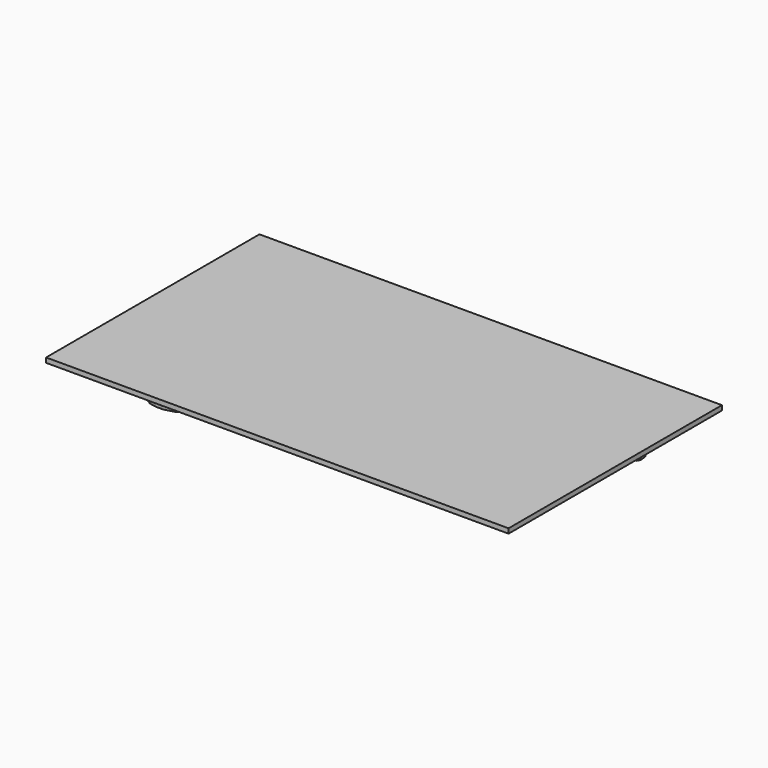
from build123d import *

# Parameters (mm, degrees)
F1_DEPTH = 2
F3_W     = 97.3806902766
F3_H     = 56.1529509723
F4_DEPTH = 1


with BuildPart() as f1:
    # F0 (on Top) → F1 (new body)
    with BuildSketch(Plane.XY):
        Polygon((23.6468666, -2.9716222), (23.3256315665, -2.7068344444), (23.2722166, -2.7745182), (23.0324406, -2.9523436), (22.6933506, -3.1164276), (22.3049846, -3.1880556), (22.1726506, -3.1880556), (21.7385646, -3.0351476), (21.4050626, -2.7651456), (21.2343746, -2.6602436), (20.8787746, -2.4037036), (20.5562335082, -2.1246834637), (20.5313026, -2.3142956), (20.5051406, -2.4204676), (20.2666346, -2.6328116), (20.1343006, -2.8172156), (19.8698866, -3.0818582), (18.9603126, -3.8385242), (17.8333146, -4.1403016), (17.7629566, -3.8880796), (17.8333146, -3.4788856), (18.0715666, -2.9233622), (18.4144666, -2.5787096), (19.4756786, -2.3211536), (20.5370916003, -2.1081244023), (20.5079346, -2.0829016), (20.2945746, -1.7849596), (20.2046131837, -1.7139919569), (19.3946526, -1.8390616), (18.9438026, -1.9973036), (18.4144666, -2.0496022), (17.9214526, -2.3005796), (17.5686466, -2.7110436), (17.2519086, -3.4527236), (17.1716446, -3.7432996), (17.2778166, -4.2464736), (17.5948086, -4.4585636), (18.0441346, -4.4806616), (18.4947306, -4.4049442), (18.5468006, -4.3785536), (19.2361566, -4.1403016), (19.6590666, -3.7694616), (19.3405506, -4.3262296), (19.0499746, -4.9078642), (18.6270646, -5.8862976), (18.5747406, -6.0983622), (18.7027566, -6.5380616), (19.0499746, -6.7598036), (19.5351146, -6.7791076), (20.0019666, -6.6015616), (20.5368906, -6.0846462), (21.1144866, -5.6493156), (21.3250526, -6.0722256), (21.4312246, -6.5477136), (21.6161366, -6.8080636), (21.8820746, -7.0506082), (22.0926406, -7.1044816), (22.7375466, -7.1623936), (23.2049066, -6.9444616), (23.3634026, -6.7074796), (23.3923586, -6.0681616), (23.3634026, -5.4892956), (23.3235246, -4.9739296), (23.2049066, -4.4585636), (23.3093006, -4.4585636), (23.8663226, -5.0925476), (23.9986566, -5.3846222), (24.8447306, -5.8862976), (25.3738126, -6.1245496), (25.5061466, -6.1783722), (25.9318506, -6.0750196), (26.2198866, -5.7539636), (26.2475726, -5.6754776), (26.1937246, -5.0262536), (25.9831586, -4.4585636), (25.6905506, -4.0313102), (25.3999746, -3.6648136), (25.1642626, -3.4816796), (25.1049691663, -3.4368495289), (24.4477286, -3.3727136), (24.3677186, -3.4527236), (24.2656106, -3.3823402), (23.9958626, -3.2129476), align=None)
        Polygon((20.4528166, -5.4892956), (20.2404726, -5.6754776), (19.9953626, -6.0282836), (19.7113906, -6.2830456), (19.1823086, -6.3368682), (19.2361566, -6.0186316), (19.8437246, -4.6955456), (20.7698086, -3.4003742), (20.9018886, -3.2045656), (21.1144866, -3.1080456), (21.0342226, -3.6373816), (20.9018886, -4.2203116), (20.7436466, -4.6432216), (20.6113126, -5.0925476), align=None, mode=Mode.SUBTRACT)
        Polygon((21.9603066, -4.4585636), (22.1726506, -3.8756082), (22.2249746, -3.5586416), (22.3832166, -3.3465516), (22.5155506, -3.4885376), (22.6478846, -3.6909756), (22.6631246, -4.1169336), (22.7497386, -4.7217076), (22.8521006, -5.3267356), (22.9125526, -5.7539636), (22.9554786, -6.0709302), (22.9402386, -6.3892176), (22.8602286, -6.5477136), (22.6577906, -6.7364102), (22.3573086, -6.7861942), (22.3311466, -6.7861942), (22.1878906, -6.5050416), (22.0664786, -6.2045596), (21.9864686, -5.4892956), (21.9082366, -4.8017176), align=None, mode=Mode.SUBTRACT)
        Polygon((24.6488966, -5.1613816), (24.1833146, -4.4585636), (24.0372646, -4.1306496), (23.8924846, -3.7432996), (23.8081566, -3.4842196), (23.7863126, -3.3465516), (23.9707166, -3.3727136), (24.1571526, -3.4003742), (24.6227346, -3.5642296), (24.9509026, -3.8494716), (25.2305566, -4.0864282), (25.4538226, -4.4049442), (25.7474466, -4.9271936), (25.7446526, -5.6493156), (25.6905506, -5.7016142), (25.2938026, -5.6493156), align=None, mode=Mode.SUBTRACT)
        Polygon((23.8233966, -2.3833836), (23.6172765796, -2.0582420765), (23.3634026, -2.6589736), (23.3256315665, -2.7068344444), (23.6468666, -2.9716222), (23.9958626, -3.2129476), (24.2656106, -3.3823402), (24.3677186, -3.4527236), (24.4477286, -3.3727136), (25.1049691663, -3.4368495289), (24.9509026, -3.3203642), (24.5800626, -3.0874716), (24.1309906, -2.8972256), (24.0509806, -2.8710636), (23.9448086, -2.7389836), align=None)
        Polygon((24.8185686, -1.4161516), (24.8035180213, -1.4201773166), (23.6539786, -1.9713956), (23.6172765796, -2.0582420765), (23.8233966, -2.3833836), (23.9448086, -2.7389836), (24.0509806, -2.8710636), (24.1309906, -2.8972256), (24.5800626, -3.0874716), (24.9509026, -3.3203642), (25.1049691663, -3.4368495289), (25.2676406, -3.4527236), (25.5582166, -3.5586416), (26.5122406, -3.3203642), (27.0413226, -3.1080456), (27.1736566, -3.0295596), (27.4065746, -2.6617422), (27.3842226, -2.2358096), (27.3583146, -2.1819616), (26.8813026, -1.7811496), (26.3260586, -1.5205456), (25.8393946, -1.4118336), (25.3738126, -1.3620496), (25.0746006, -1.3785596), align=None)
        Polygon((25.8863846, -2.9592016), (25.0570746, -2.7910536), (24.7344946, -2.6645616), (24.3956586, -2.5004776), (24.1528346, -2.3734776), (24.0509806, -2.2881082), (24.1833146, -2.1819616), (24.3153946, -2.0775676), (24.7507506, -1.8679922), (25.1894086, -1.8390616), (25.5488186, -1.8016982), (25.9290566, -1.8652236), (26.5107166, -2.0402042), (27.0136366, -2.5528016), (27.0136366, -2.6328116), (26.6966446, -2.8710636), align=None, mode=Mode.SUBTRACT)
        Polygon((25.1091446, 1.3359384), (24.5000526, 0.9130284), (24.2714526, 0.6592824), (24.0248186, 0.4639564), (24.1007646, 0.7517638), (24.1571526, 1.0974324), (24.2633246, 1.7329404), (24.3956586, 2.7911044), (24.3956586, 3.0034484), (24.1556286, 3.3948624), (23.7601506, 3.5066478), (23.2831386, 3.3839404), (22.8863906, 3.0819344), (22.5282506, 2.4550624), (22.0926406, 1.8650204), (21.7759026, 2.2096984), (21.5373966, 2.6328878), (21.2988906, 2.8353004), (20.9821526, 2.9775404), (20.7698086, 2.9775404), (20.1579226, 2.8726384), (19.7652386, 2.5266904), (19.6852286, 2.2358858), (19.8465186, 1.6255238), (20.0299066, 1.0712704), (20.2239626, 0.5864098), (20.4789786, 0.1192784), (20.3728066, 0.0931418), (19.6852286, 0.5421884), (19.4728846, 0.7806944), (18.5206386, 1.0192004), (17.9653946, 1.0974324), (17.8333146, 1.0974324), (17.4652686, 0.8840724), (17.2778166, 0.4901438), (17.2778166, 0.4098544), (17.5216566, -0.1812036), (17.8853846, -0.6744716), (18.2684166, -1.0079482), (18.6529726, -1.2838176), (18.9275466, -1.3981176), (19.1823086, -1.4943582), (19.6014086, -1.6170656), (20.0822306, -1.6805656), (20.1622406, -1.6805656), (20.2046131837, -1.7139919569), (20.7698086, -1.6267176), (21.2465666, -1.0453116), (21.3679786, -0.9584436), (21.6489026, -0.8591296), (22.0194886, -0.7986522), (22.4111566, -0.8329676), (22.5434906, -0.8591296), (22.9153466, -1.1334496), (23.0297911258, -1.2959904244), (23.2435146, -1.3691616), (23.4154726, -1.6805656), (23.4154726, -1.7328642), (23.4089527537, -1.7725239478), (23.4243429347, -1.7923627405), (23.7063026, -1.7067276), (23.8924846, -1.7328642), (23.9448086, -1.7067276), (24.3913406, -1.5304262), (24.8035180213, -1.4201773166), (24.9247406, -1.3620496), (25.3214886, -1.0714736), (25.8228846, -0.8591296), (26.2391906, -0.4814316), (26.4581386, 0.0131318), (26.5645646, 0.8068818), (26.5645646, 1.1253978), (26.3260586, 1.5744444), (25.9831586, 1.6806418), (25.5378966, 1.5716504), (25.1353066, 1.3621258), align=None)
        Polygon((19.0073026, 0.3715004), (19.6590666, -0.1715516), (19.8863966, -0.4483862), (20.1343006, -0.8068056), (20.2902566, -1.0288016), (20.3466446, -1.1514836), (20.1622406, -1.1776456), (19.9760586, -1.2035536), (19.4993006, -1.1761216), (19.1038226, -0.9912096), (18.7649866, -0.8428736), (18.4685686, -0.5944616), (18.0304186, -0.1784096), (17.8333146, 0.5160264), (17.8592226, 0.5962904), (18.2562246, 0.6745224), align=None, mode=Mode.SUBTRACT)
        Polygon((23.9186466, -0.8068056), (23.9986566, -0.5944616), (24.1833146, -0.2777236), (24.4766846, 0.2348484), (24.8239026, 0.7047484), (25.2610366, 1.0811764), (25.8228846, 1.3097764), (25.9552186, 1.1017504), (26.0090666, 0.6745224), (25.9290566, 0.0669544), (25.8091686, -0.1646936), (25.6905506, -0.3577336), (24.7355106, -0.9058656), (23.7601506, -1.4161516), (23.7339886, -1.2035536), (23.7339886, -1.0973562), align=None, mode=Mode.SUBTRACT)
        Polygon((21.7759026, 0.4639564), (21.7497406, -0.1715516), (21.7759026, -0.4900676), (21.6697306, -0.7267956), (21.5165686, -0.6373876), (21.3250526, -0.4900676), (21.1774786, -0.0831596), (20.9214466, 0.4733544), (20.6555086, 1.0258044), (20.4789786, 1.4159484), (20.2666346, 2.0235164), (20.2945746, 2.2096984), (20.4350366, 2.4781764), (20.7174846, 2.6067004), (20.7436466, 2.6067004), (20.9653886, 2.3654004), (21.1665566, 2.1035264), (21.4573866, 1.4421358), (21.7497406, 0.8068818), align=None, mode=Mode.SUBTRACT)
        Polygon((22.9664006, 1.8650204), (23.0987346, 2.1035264), (23.2239566, 2.5142444), (23.4695746, 2.8452064), (23.9707166, 3.0557724), (23.9986566, 2.7390344), (23.7863126, 1.3097764), (23.2572306, -0.1974596), (23.1977946, -0.4346956), (23.0187246, -0.5944616), (22.9402386, -0.0653796), (22.9125526, 0.5421884), (22.9402386, 0.9930384), (22.9402386, 1.4421358), align=None, mode=Mode.SUBTRACT)
        Polygon((23.2722166, -2.7745182), (23.3256315665, -2.7068344444), (23.3026966, -2.6879296), (23.0504746, -2.3899876), (23.0483140565, -2.3818247273), (22.9125526, -2.4743156), (22.4893886, -2.8710636), (22.3268286, -2.7209496), (22.1464886, -2.5528016), (21.9603066, -2.5004776), (21.5635586, -2.2317456), (21.3250526, -1.7067276), (21.2988906, -1.4682216), (21.4007446, -1.3264642), (21.5635586, -1.2838176), (21.9892626, -1.3648436), (22.2788226, -1.6267176), (22.3476566, -1.9010376), (22.4373186, -2.0775676), (22.4893886, -2.0661376), (22.5434906, -1.9172936), (22.5434906, -1.6805656), (22.5696526, -1.4682216), (22.9125526, -1.2558522), (23.0297911258, -1.2959904244), (22.9153466, -1.1334496), (22.5434906, -0.8591296), (22.4111566, -0.8329676), (22.0194886, -0.7986522), (21.6489026, -0.8591296), (21.3679786, -0.9584436), (21.2465666, -1.0453116), (20.7698086, -1.6267176), (20.2046131837, -1.7139919569), (20.2945746, -1.7849596), (20.5079346, -2.0829016), (20.5370916003, -2.1081244023), (20.5589886, -2.1037296), (20.5562335082, -2.1246834637), (20.8787746, -2.4037036), (21.2343746, -2.6602436), (21.4050626, -2.7651456), (21.7385646, -3.0351476), (22.1726506, -3.1880556), (22.3049846, -3.1880556), (22.6933506, -3.1164276), (23.0324406, -2.9523436), align=None)
        Polygon((23.3634026, -2.6589736), (23.6172765796, -2.0582420765), (23.5577126, -1.9642836), (23.4243429347, -1.7923627405), (23.404711171, -1.7983251849), (23.3634026, -2.0496022), (23.1675686, -2.3005796), (23.0483140565, -2.3818247273), (23.0504746, -2.3899876), (23.3026966, -2.6879296), (23.3256315665, -2.7068344444), align=None)
        Polygon((23.6539786, -1.9713956), (24.8035180213, -1.4201773166), (24.3913406, -1.5304262), (23.9448086, -1.7067276), (23.8924846, -1.7328642), (23.7063026, -1.7067276), (23.4243429347, -1.7923627405), (23.5577126, -1.9642836), (23.6172765796, -2.0582420765), align=None)
    extrude(amount=F1_DEPTH)



with BuildPart() as f1b:
    # F0 (on Top) → F1, piece 2 (new body)
    with BuildSketch(Plane.XY):
        Polygon((-19.2621154, 3.0766004), (-19.4208654, 2.8452064), (-19.4208654, 2.8172664), (-19.2346834, 2.5525984), (-18.9438534, 2.5266904), (-18.5991754, 2.5266904), (-18.1501034, 2.3681944), (-18.1501034, -0.4621022), (-18.1762654, -1.0453116), (-18.1762654, -1.1514836), (-18.1501034, -1.3620496), (-18.1762654, -1.7328642), (-18.2024274, -2.7651456), (-18.2024274, -4.6170596), (-18.3085994, -5.1461416), (-18.3886094, -5.7278016), (-18.4947814, -6.8398136), (-18.4668414, -7.1306182), (-18.4668414, -7.2091296), (-18.5471054, -7.6858622), (-18.7053474, -8.7181182), (-18.8638434, -9.7503742), (-19.3146934, -11.2317276), (-19.7114414, -12.1039636), (-20.0822814, -13.0299968), (-20.4513434, -13.5068056), (-21.1859114, -14.3391382), (-22.1188534, -14.935835), (-22.7182934, -15.0667466), (-23.3357674, -15.120493), (-23.9875314, -15.047468), (-24.5801134, -14.935835), (-24.8709434, -14.74978), (-25.2415294, -14.6450812), (-25.5323594, -14.4328388), (-26.1978394, -13.8967972), (-26.7228574, -13.2422138), (-27.5689314, -11.4699796), (-27.7274274, -10.7285536), (-28.0721054, -9.2995496), (-28.1518614, -8.5596222), (-28.2567634, -8.0828642), (-28.2841954, -7.4476356), (-28.2841954, -6.8123816), (-28.2041854, -5.5693056), (-28.1244294, -1.6267176), (-28.2041854, -0.3297936), (-28.2306014, 0.1992884), (-28.1244294, 2.2358858), (-28.0197814, 2.2358858), (-27.5663914, 2.3463504), (-27.3306794, 2.6328878), (-27.5950934, 2.9775404), (-28.1518614, 3.0034484), (-30.1886874, 3.0819344), (-30.7949854, 3.0296358), (-31.0624474, 2.7390344), (-31.0624474, 2.7128978), (-30.9329074, 2.5295098), (-30.6585874, 2.4715724), (-30.3555654, 2.4482044), (-30.1363634, 2.3681944), (-30.0301914, 1.9714464), (-30.1086774, 1.0453878), (-30.1363634, -0.2515616), (-30.1363634, -2.1037296), (-30.1625254, -4.3262296), (-30.1625254, -4.5908722), (-30.0563534, -5.5954676), (-29.9763434, -6.9721222), (-29.9501814, -7.6597256), (-29.9763434, -8.2413856), (-29.9763434, -8.3998816), (-29.8181014, -9.4057216), (-29.4472614, -11.3640616), (-29.3261034, -11.8187216), (-29.1041074, -12.2362976), (-28.7238694, -13.01623), (-28.2841954, -13.719048), (-27.9920954, -14.0621512), (-27.7274274, -14.4066768), (-27.2920714, -14.8393404), (-26.7751814, -15.1742394), (-26.4322814, -15.3588974), (-25.6591054, -15.67307), (-24.8447814, -15.8880556), (-24.7386094, -15.914243), (-23.8125254, -16.100298), (-23.4681014, -16.12646), (-22.7802694, -16.0203388), (-22.6743514, -15.9941768), (-22.0926914, -15.8357062), (-21.0865974, -15.4649932), (-20.1346054, -15.0143718), (-19.7376034, -14.74978), (-19.3408554, -14.4590262), (-19.0500254, -13.7975594), (-18.7053474, -13.16228), (-18.8638434, -16.2325812), (-18.9367414, -17.752568), (-19.2085214, -19.115405), (-20.8221834, -19.115405), (-21.4574374, -19.089243), (-22.2773494, -19.0630556), (-23.0972614, -19.089243), (-24.6585994, -19.1953388), (-25.4000254, -19.3538094), (-26.1676134, -19.4337432), (-26.6966954, -19.6445632), (-27.1721834, -19.8568056), (-28.2041854, -20.5444344), (-28.3103574, -20.6243682), (-28.4165294, -20.7304894), (-28.6273494, -20.9413094), (-28.8135314, -21.1535518), (-29.0243514, -21.3643718), (-29.2102794, -21.7350594), (-29.5795954, -22.4226882), (-29.7462194, -22.8058218), (-29.8716954, -23.27021), (-29.9501814, -23.9578388), (-29.9501814, -24.6992394), (-29.7916854, -24.9899932), (-29.7119294, -25.3331218), (-29.3784274, -25.8553966), (-29.0243514, -26.3390634), (-28.5750254, -26.7883132), (-28.1780234, -27.0005556), (-27.8447754, -27.1755616), (-27.4904454, -27.2913094), (-26.4846054, -27.4773644), (-25.2938534, -27.5035518), (-25.0030234, -27.5035518), (-24.3677694, -27.3974306), (-23.1511094, -27.052905), (-22.5681794, -26.8682724), (-21.1668614, -25.9945632), (-20.7160114, -25.625298), (-20.3469494, -25.1484638), (-20.0022714, -24.671655), (-19.3146934, -23.667085), (-19.1561974, -23.2233724), (-18.9176914, -22.8195632), (-18.7053474, -22.079585), (-18.6271154, -21.8149932), (-18.4147714, -21.5242394), (-18.2562754, -21.1535518), (-17.9918614, -19.7768718), (-16.5105334, -19.7506844), (-14.5260314, -19.7768718), (-13.4676134, -19.8044562), (-11.3230914, -19.6445632), (-10.9801914, -19.6445632), (-9.6573594, -19.5660518), (-7.9113634, -19.486118), (-6.7729354, -19.3276474), (-5.6347614, -19.1691768), (-5.1595274, -19.0630556), (-4.6301914, -18.904585), (-2.5659334, -18.4277762), (-0.4752594, -17.9785518), (0.5831586, -17.7924968), (2.4612346, -17.13103), (3.4655506, -16.8664382), (4.8686466, -16.311118), (5.3456586, -16.1526474), (6.2176406, -15.6234638), (7.1437246, -15.1742394), (8.3883246, -14.352905), (9.1279726, -13.8237468), (10.8739686, -12.4222256), (11.1386366, -12.1578116), (11.3248186, -11.7869716), (11.6153946, -11.4961416), (11.9062246, -11.1517176), (12.1968006, -10.8608622), (12.9643886, -9.8027236), (13.5198866, -9.1108022), (13.9966446, -8.3211416), (14.3413226, -7.4737976), (14.7340066, -6.5641982), (15.0289006, -5.6754776), (15.2935686, -3.6111942), (15.2674066, -2.9495496), (14.8965666, -1.4682216), (14.0228066, 0.1192784), (13.6799066, 0.3839464), (13.5737346, 0.5683758), (12.7538226, 1.3359384), (12.0123966, 1.8129504), (11.1663226, 2.2096984), (10.2402386, 2.3943818), (9.5511366, 2.4743918), (8.2559906, 2.2881844), (7.4510646, 2.0153884), (6.8269866, 1.6006318), (6.2976506, 1.0192004), (6.0070746, 0.1992884), (5.9791346, -0.0653796), (6.0809886, -0.6940296), (6.3238126, -1.2838176), (6.8434966, -1.7219676), (7.5404726, -2.0234656), (8.0174846, -2.0496022), (8.2280506, -2.0496022), (8.7548466, -1.8512536), (9.1820746, -1.5743682), (9.2603066, -1.4943582), (9.5249746, -0.8329676), (9.4050866, -0.2995676), (9.1279726, 0.0931418), (8.5988906, 0.2775204), (8.5206586, 0.2775204), (8.2186526, 0.0738124), (7.9374746, -0.2515616), (7.4884026, -0.4621022), (7.2237346, -0.4359656), (7.1975726, -0.1715516), (7.2237346, 0.3839464), (7.5145646, 0.9391904), (7.8851506, 1.2036044), (8.5755226, 1.4601444), (9.3664786, 1.5744444), (9.5788226, 1.5744444), (10.5267506, 1.4655038), (11.3768886, 1.1776964), (12.3291346, 0.5962904), (12.8089406, 0.2348484), (13.1508246, -0.2253742), (13.2925566, -0.8052816), (13.3352286, -1.4682216), (13.4414006, -2.6066242), (13.4414006, -2.8172156), (13.3352286, -3.4003742), (13.3090666, -4.0341296), (13.0967226, -4.7232316), (12.9123186, -5.4108096), (12.4614686, -6.8398136), (12.1279666, -7.6528676), (11.6956586, -8.3473036), (11.4833146, -8.6119716), (10.9237526, -9.4250002), (10.3448866, -10.1994716), (9.4188026, -11.1255556), (7.9113126, -12.4222256), (7.4343006, -12.8191768), (6.3761366, -13.5867394), (5.3177186, -14.352905), (4.1602406, -15.0336758), (2.9644086, -15.6758132), (1.7198086, -16.2587432), (0.4228846, -16.8140888), (-0.2105914, -17.1586144), (-0.9357614, -17.3763432), (-1.6398494, -17.5554894), (-2.3012654, -17.7663094), (-3.2273494, -17.8724306), (-4.1011094, -18.0570632), (-6.0053474, -18.3492394), (-7.8051914, -18.692368), (-10.2126034, -18.878423), (-11.8674134, -18.940399), (-13.6784334, -18.9831218), (-14.0231114, -18.9831218), (-17.3042834, -18.8246512), (-17.8333654, -18.8246512), (-17.7010314, -17.4879762), (-17.5686974, -15.9941768), (-17.5410114, -14.9881844), (-17.4625254, -14.0359638), (-17.4625254, -13.8237468), (-17.4886874, -12.9776474), (-17.4625254, -12.0254776), (-17.5410114, -11.0732316), (-17.5148494, -9.9348036), (-17.6730914, -8.9289636), (-17.5948594, -7.8705456), (-17.6730914, -6.7598036), (-17.6730914, -6.2045596), (-17.5148494, -2.0234656), (-17.3301914, 0.2516378), (-17.2585634, 1.4159484), (-17.1440094, 2.5805384), (-16.4043614, 2.7651964), (-16.0335214, 2.8713938), (-15.9273494, 3.1357824), (-15.9273494, 3.2142684), (-16.1917634, 3.3742884), (-16.7749474, 3.2681418), (-17.0396154, 3.2681418), (-18.0523134, 3.3478724), (-18.9438534, 3.4266378), align=None)
        Polygon((-25.9814314, -26.7359384), (-26.6431014, -26.6036806), (-26.8290294, -26.4975594), (-27.0936974, -26.419048), (-27.4904454, -26.1268718), (-27.8915114, -25.8788408), (-28.2306014, -25.5715262), (-28.4426914, -24.5669562), (-28.3710634, -23.80488), (-28.1780234, -23.1640888), (-27.7274274, -22.3441768), (-27.1721834, -21.656548), (-26.5369294, -21.285835), (-25.5158494, -20.8310734), (-24.3154454, -20.5182724), (-22.5681794, -20.2274932), (-20.9021934, -19.882993), (-19.8437754, -19.8044562), (-19.6575934, -19.7768718), (-19.3667634, -19.882993), (-19.5531994, -20.7553052), (-19.8960994, -21.5504268), (-20.5575154, -22.847173), (-21.3251034, -23.9578388), (-22.0665294, -24.8838974), (-22.5158554, -25.2807724), (-22.9649274, -25.6514346), (-23.6001814, -26.022173), (-24.2354354, -26.3652762), (-24.6847614, -26.4713974), align=None, mode=Mode.SUBTRACT)
    extrude(amount=F1_DEPTH)


with BuildPart() as f1c:
    # F0 (on Top) → F1, piece 3 (new body)
    with BuildSketch(Plane.XY):
        Polygon((-11.6484654, 3.0075124), (-12.1709434, 2.8452064), (-12.9385314, 2.3420324), (-13.4676134, 1.7867884), (-14.0231114, 0.9130284), (-14.3398494, 0.2775204), (-14.6583654, -0.3297936), (-15.1335994, -1.7590516), (-15.3197814, -2.5266142), (-15.4782774, -3.3203642), (-15.5565094, -4.1141142), (-15.6888434, -4.8555656), (-15.7426914, -5.6754776), (-15.7950154, -6.4953642), (-15.8488634, -7.7920596), (-15.7426914, -9.8550476), (-15.6365194, -10.6226356), (-15.2918414, -12.0254776), (-15.0012654, -12.6330456), (-14.6845274, -13.1898644), (-13.8366754, -14.0883132), (-13.1229354, -14.512798), (-12.1447814, -14.6450812), (-11.6677694, -14.6174968), (-11.0063534, -14.4590262), (-10.3710994, -14.3005556), (-9.8679254, -13.8774932), (-9.4188534, -13.4268718), (-9.1282774, -12.95146), (-9.0221054, -12.7929894), (-8.6774274, -12.0778016), (-8.3604354, -11.3378742), (-8.0698594, -10.5441242), (-7.9375254, -9.9348036), (-7.7792834, -9.3257116), (-7.7251814, -8.8243156), (-7.6190094, -8.3473036), (-7.5666854, -7.8443582), (-7.4866754, -7.3691242), (-7.4866754, -6.5215516), (-7.4084434, -6.1783722), (-7.3822814, -5.7816242), (-7.3022714, -5.0140616), (-7.4881994, -3.0983936), (-7.8313534, -1.3620496), (-8.1760314, -0.2777236), (-8.2021934, -0.1974596), (-8.3865974, 0.3316478), (-8.7835994, 1.3621258), (-9.2865194, 2.1296884), (-9.8100134, 2.6536904), (-10.5293414, 2.9775404), (-11.0063534, 3.0296358), align=None)
        Polygon((-11.7480334, -13.95603), (-12.0386094, -14.0359638), (-12.3596654, -13.8761216), (-12.6200154, -13.6390888), (-12.8323594, -13.4544562), (-13.3876034, -12.7130556), (-13.7322814, -12.2362976), (-13.8646154, -11.8392956), (-13.9969494, -11.4961416), (-14.0751814, -11.0455456), (-14.2613634, -9.7227136), (-14.3660114, -8.3473036), (-14.3936974, -7.8705456), (-14.3660114, -6.9444616), (-14.3136874, -6.0460636), (-14.1813534, -5.1461416), (-14.0751814, -4.5108622), (-13.9969494, -4.0618156), (-13.7846054, -3.0557216), (-13.5199374, -1.7590516), (-13.3075934, -0.9653016), (-12.7785114, 0.5421884), (-12.4356114, 1.2577064), (-12.1168414, 1.9973544), (-11.6939314, 2.3681944), (-11.0325154, 2.6587704), (-10.6896154, 2.6587704), (-10.2141274, 2.3791164), (-9.8158554, 1.9191478), (-9.4188534, 1.0712704), (-9.1282774, 0.0931418), (-8.7574374, -1.4420596), (-8.7051134, -1.9713956), (-8.5450934, -2.5528016), (-8.5450934, -2.8972256), (-8.5189314, -3.2142176), (-8.4406994, -3.7694616), (-8.4406994, -4.3785536), (-8.3604354, -4.9340516), (-8.3604354, -5.0925476), (-8.3865974, -5.7278016), (-8.3865974, -5.8862976), (-8.3604354, -6.5215516), (-8.3865974, -7.0767956), (-8.4127594, -7.6335636), (-8.4127594, -8.1628742), (-8.7312754, -10.7285536), (-8.7835994, -11.2317276), (-9.1541854, -12.1039636), (-9.2065094, -12.1839736), (-9.7096834, -13.0575812), (-10.1064314, -13.4268718), (-10.5293414, -13.7713974), (-11.0505494, -13.8926824), align=None, mode=Mode.SUBTRACT)
    extrude(amount=F1_DEPTH)


with BuildPart() as f1d:
    # F0 (on Top) → F1, piece 4 (new body)
    with BuildSketch(Plane.XY):
        Polygon((-1.1105134, 3.5066478), (-1.1105134, 3.3463484), (-1.4165834, 3.2719264), (-1.5613634, 3.0557724), (-1.4691614, 2.8683204), (-1.2166854, 2.8172664), (-0.7676134, 2.8452064), (-0.6876034, 2.8452064), (-0.6876034, 2.5805384), (-0.7676134, 1.0453878), (-0.7937754, 0.3839464), (-0.7676134, -0.9653016), (-0.7676134, -5.7539636), (-0.8199374, -6.3892176), (-0.7676134, -7.7120496), (-0.7137654, -8.3473036), (-0.6614414, -8.9828116), (-0.6614414, -9.6442276), (-0.5814314, -10.3841296), (-0.5293614, -11.2055656), (-0.6355334, -12.0254776), (-0.8199374, -12.5007116), (-1.0195814, -12.8908302), (-1.2969494, -13.16228), (-1.3231114, -13.1898644), (-1.7980914, -13.559155), (-2.1950934, -13.6129268), (-2.5918414, -13.6652762), (-2.8565094, -13.6390888), (-3.1211774, -13.559155), (-3.4699194, -13.2904484), (-3.5979354, -12.8453388), (-3.7043614, -12.4483622), (-3.7302694, -12.2362976), (-3.7302694, -11.9993156), (-3.7564314, -11.8131082), (-3.7564314, -11.6023136), (-3.8364414, -11.2840516), (-3.8364414, -10.9932216), (-3.8626034, -10.8347256), (-3.8626034, -10.6762296), (-3.9949374, -9.9611942), (-4.0472614, -8.6919816), (-4.1534334, -8.0567276), (-4.1534334, -7.1568056), (-4.1793414, -6.2568582), (-4.2334434, -2.7389836), (-4.3116754, -1.0714736), (-4.2855134, -0.7544816), (-4.3396154, 0.2516378), (-4.3657774, 0.5160264), (-4.3657774, 0.7806944), (-4.4178474, 1.2838938), (-4.3657774, 1.5744444), (-4.3657774, 1.7329404), (-4.3396154, 1.8650204), (-4.2334434, 2.4743918), (-3.9855394, 2.6963624), (-3.5979354, 2.8172664), (-3.3073594, 2.8172664), (-3.0950154, 3.0034484), (-3.2055054, 3.2061658), (-3.4917634, 3.2681418), (-4.2334434, 3.1881318), (-4.5501814, 3.2681418), (-4.6042834, 3.2681418), (-4.8948594, 3.2419544), (-4.9210214, 3.2942784), (-5.0792634, 3.3204404), (-5.6624474, 3.2419544), (-6.3761874, 3.1096204), (-6.6667634, 3.1357824), (-6.9052694, 2.9775404), (-6.9052694, 2.9496258), (-6.6944494, 2.7664664), (-6.2438534, 2.7390344), (-5.7947814, 2.7128978), (-5.7409334, 2.3943818), (-5.7668414, 1.9191478), (-5.7668414, 1.7867884), (-5.6886094, 1.3900404), (-5.6886094, 1.1776964), (-5.7409334, 0.1454404), (-5.7409334, -0.1192276), (-5.7147714, -1.0453116), (-5.7147714, -1.2297156), (-5.7668414, -2.1819616), (-5.7668414, -2.3943056), (-5.7147714, -2.7910536), (-5.7147714, -3.8233096), (-5.6624474, -4.3785536), (-5.6624474, -4.5632116), (-5.6886094, -5.4108096), (-5.6624474, -6.4692276), (-5.6886094, -8.6381082), (-5.6886094, -10.6487976), (-5.6266334, -11.7044216), (-5.4239414, -12.6607316), (-5.2656994, -13.136118), (-5.0792634, -13.6129268), (-4.6896274, -13.9891262), (-4.1011094, -14.1682724), (-3.6240974, -14.2206218), (-3.2811974, -14.2482062), (-2.5397714, -14.1682724), (-2.1689314, -14.0883132), (-1.7198594, -13.929868), (-1.2428474, -13.5867394), (-1.0322814, -13.3745224), (-0.8806434, -13.1057904), (-0.6876034, -12.8976882), (-0.3970274, -12.4222256), (-0.3167634, -12.8191768), (-0.0523494, -13.4806182), (0.1117346, -13.6418574), (0.2384806, -13.8237468), (0.7330186, -14.131036), (1.3489686, -14.3005556), (1.5351506, -14.3005556), (2.0103846, -14.142085), (2.5135586, -13.95603), (2.7779726, -13.8237468), (3.0426406, -13.6652762), (3.2288226, -13.2945632), (3.3873186, -12.8715262), (3.4134806, -12.6607316), (3.3611566, -12.4222256), (3.0164786, -12.2898916), (2.8320746, -12.3160536), (2.3217886, -12.4704856), (2.0903946, -12.8453388), (2.0903946, -13.2160518), (1.9651726, -13.5756904), (1.7198086, -13.7975594), (1.3850366, -13.6845802), (1.1122406, -13.4544562), (0.9799066, -13.1898644), (0.8475726, -12.925298), (0.7414006, -12.6068582), (0.6090666, -12.3160536), (0.5552186, -11.9454676), (0.3446526, -11.2840516), (0.3446526, -10.8870496), (0.3184906, -10.4903016), (0.3184906, -10.3579676), (0.3446526, -9.7227136), (0.3184906, -9.1410536), (0.2905506, -8.8243156), (0.3184906, -8.5057996), (0.2643886, -7.3414636), (0.2643886, -7.0767956), (0.3446526, -5.1461416), (0.2905506, -2.8172156), (0.2123186, -1.6528796), (0.2123186, 0.4639564), (0.3184906, 1.2036044), (0.3184906, 1.6806418), (0.3446526, 2.1558758), (0.4561586, 2.6110184), (0.6875526, 2.9234384), (1.0652506, 3.0143704), (1.3228066, 3.2419544), (1.3228066, 3.2942784), (1.1368786, 3.4004504), (0.7937246, 3.4266378), (0.1861566, 3.4004504), (-0.9784334, 3.5066478), align=None)
    extrude(amount=F1_DEPTH)


with BuildPart() as f1e:
    # F0 (on Top) → F1, piece 5 (new body)
    with BuildSketch(Plane.XY):
        Polygon((-1.2969494, 24.1703098), (-1.5371687202, 24.3378402769), (-1.2166854, 24.0641124), (-0.8722614, 23.6671358), (-0.4752594, 23.1118664), (-0.3774694, 22.7382324), (-0.3167634, 22.2642938), (-0.2908554, 21.3658704), (-0.2385314, 19.5660518), (-0.2385314, 17.7141124), (-0.1846834, 16.8141904), (-0.1846834, 15.8619444), (-0.0785114, 14.6973544), (-0.0785114, 13.5330438), (-0.0523494, 12.3161044), (-0.0785114, 9.9089464), (-0.0523494, 8.8243918), (-0.0785114, 7.6597764), (-0.0785114, 7.6338938), (-0.1361694, 7.0425564), (-0.2908554, 6.6275204), (-0.5814314, 6.4692784), (-1.1105134, 6.3369444), (-1.2166854, 6.3369444), (-1.7460214, 6.4692784), (-2.0627594, 6.4692784), (-2.2751034, 6.4954404), (-2.3274274, 6.4954404), (-2.7241754, 6.2846204), (-2.6058114, 6.0529724), (-2.4074374, 5.7817004), (-2.2489414, 5.3750464), (-1.8521934, 5.2264564), (-1.2428474, 5.3587904), (-0.7676134, 5.3587904), (0.2123186, 5.3846984), (0.8998966, 5.3846984), (1.6936466, 5.4108858), (2.3027386, 5.3587904), (2.9364686, 5.3046884), (3.1226506, 5.1723544), (3.3611566, 5.1202844), (3.7040566, 5.2785264), (3.7302186, 5.4108858), (3.5978846, 5.9140344), (3.5978846, 5.9661044), (3.6258246, 6.3107824), (3.5788346, 6.6224404), (3.4134806, 6.8139564), (3.3611566, 6.8139564), (2.9644086, 6.6536824), (2.6415746, 6.5683384), (2.3027386, 6.5213484), (2.2488906, 6.5213484), (1.9321526, 6.7339464), (1.7888966, 6.9196204), (1.7457166, 7.1830184), (1.6413226, 7.4753978), (1.6674846, 7.6859384), (1.6674846, 8.3473544), (1.7198086, 8.7982044), (1.6936466, 9.2996258), (1.7198086, 9.8286824), (1.6674846, 11.0194344), (1.6936466, 11.3900204), (1.7998186, 11.8408704), (1.7998186, 12.5025404), (1.9059906, 13.0036824), (1.7998186, 13.4806944), (1.8518886, 13.9577064), (1.7998186, 14.8558504), (1.7998186, 17.6079404), (1.9321526, 18.1631844), (1.8780506, 18.5337704), (1.8780506, 19.2493138), (1.8259806, 19.5660518), (1.9044666, 20.0331324), (1.9842226, 20.4400404), (1.8259806, 20.9411824), (1.8518886, 21.0735164), (2.3507446, 20.6216758), (2.7520646, 20.0692004), (3.1226506, 19.5660518), (3.4934906, 19.0631318), (3.8363906, 18.5078624), (4.3395646, 18.0587904), (4.4457366, 17.8464464), (4.6301406, 17.6338484), (5.1853846, 16.7618664), (5.5300626, 16.3651438), (5.9009026, 15.6496004), (6.1394086, 15.3328624), (6.5884806, 14.6714464), (6.7728846, 14.3267938), (7.2498966, 13.6650984), (7.6207366, 12.8192784), (7.8313026, 12.4222764), (8.0698086, 12.0516904), (8.1759806, 11.6808758), (8.2821526, 11.5223544), (8.4665566, 11.0194344), (8.6250526, 10.6503978), (8.8373966, 10.3056944), (9.0245946, 9.8660458), (9.2341446, 9.4057724), (9.4726506, 8.6920324), (10.0802186, 7.3692004), (10.2651306, 7.0054724), (10.3725726, 6.6816478), (10.2592886, 6.4238124), (10.0278946, 6.2846204), (9.6573086, 6.2846204), (9.4988126, 6.2569344), (9.2796106, 6.1258704), (9.1820746, 5.9140344), (9.1820746, 5.8599324), (9.3403166, 5.7555384), (9.4726506, 5.7555384), (10.5310686, 5.5693818), (11.3248186, 5.5170324), (12.0385586, 5.6493918), (12.5938026, 5.6493918), (12.9123186, 5.5431944), (13.2290566, 5.5431944), (13.5737346, 5.4108858), (13.7322306, 5.5431944), (13.7581386, 5.6755284), (13.6425686, 5.9112404), (13.4675626, 6.0463938), (13.1769866, 6.7598544), (13.0708146, 6.9983858), (13.0967226, 7.3953878), (12.9643886, 8.4796884), (12.9123186, 9.0087704), (12.8582166, 9.4857824), (12.8582166, 9.5919544), (12.8861566, 10.1471984), (12.8582166, 10.3857044), (12.7261366, 10.7026964), (12.7799846, 11.1517684), (12.8061466, 11.4964464), (12.6738126, 12.6869444), (12.5676406, 13.4806944), (12.5153166, 14.0359638), (12.4091446, 14.6973544), (12.3570746, 15.1482298), (12.1706386, 17.0003978), (11.9862346, 18.8246004), (11.9323866, 20.9150204), (11.9323866, 22.4243138), (11.8800626, 23.5609638), (11.9090186, 23.9483138), (12.0385586, 24.1964464), (12.4424186, 24.3092224), (12.9702306, 24.3191284), (13.4292086, 24.3948204), (13.6260586, 24.6993664), (13.6260586, 24.7516904), (13.5008366, 24.9516138), (13.2552186, 24.9901964), (12.7799846, 24.9640598), (12.1185686, 24.9640598), (11.5092226, 25.0161044), (10.8739686, 24.9640598), (10.2925626, 24.9640598), (9.8155506, 24.9099324), (8.8112346, 24.8578624), (8.5727286, 24.6193818), (8.8112346, 24.3808504), (9.2864686, 24.3808504), (9.7893886, 24.2223544), (10.1066346, 24.1867944), (10.3448866, 24.0900204), (10.2925626, 22.3704404), (10.2925626, 22.0796358), (10.3987346, 21.0735164), (10.4248966, 20.0692004), (10.5831386, 18.1370478), (10.6093006, 17.1047664), (10.7416346, 16.2066478), (10.9278166, 14.1944344), (11.0863126, 12.1837704), (11.3768886, 8.2150204), (11.0863126, 8.0567784), (10.9801406, 8.0829404), (10.8478066, 8.2828638), (10.7957366, 8.5596984), (10.6895646, 8.7443818), (10.4510586, 9.2213938), (10.2125526, 10.0151438), (9.6049846, 11.4161824), (9.3664786, 12.1317004), (8.9557606, 12.9983484), (8.5465666, 13.8253978), (8.0957166, 14.8837904), (7.7789786, 15.5713938), (7.0652386, 16.8680638), (6.6946526, 17.5017938), (6.5361566, 17.8203098), (5.5039006, 19.3536824), (5.1333146, 19.9891904), (4.7363126, 20.5982824), (3.9164006, 21.7628978), (2.4873966, 23.3224324), (1.9842226, 23.8517938), (0.9054846, 24.7296178), (-0.2105914, 25.3869444), (-0.3970274, 25.4669798), (-0.5165411483, 25.3579435852), (0.2643886, 24.9901964), (-1.0043414, 23.9838484), align=None)
        Polygon((-1.5371687202, 24.3378402769), (-1.5875254, 24.3808504), (-0.5165411483, 25.3579435852), (-1.0846054, 25.6254504), (-1.6136874, 25.7578098), (-1.7198594, 25.7578098), (-1.7198594, 25.6775204), (-2.3576534, 25.5993138), (-2.9365194, 25.4392938), (-3.3596834, 25.3069344), (-3.7043614, 25.0963938), (-4.6042834, 24.4608858), (-4.9730914, 24.1441478), (-5.2377594, 23.7471204), (-5.3700934, 23.5609638), (-5.4762654, 23.3503978), (-5.7668414, 22.3963484), (-5.9271154, 22.3442784), (-6.3761874, 22.4766124), (-6.5885314, 22.5025204), (-7.3822814, 22.8733858), (-7.7251814, 23.2962704), (-7.8836774, 23.7194344), (-7.9375254, 23.8517938), (-7.9375254, 24.0118138), (-7.9636874, 24.1441478), (-7.7792834, 24.3547138), (-7.5407774, 24.2764564), (-7.3253854, 24.0118138), (-7.0899274, 23.7471204), (-6.8531994, 23.6932978), (-6.6146934, 23.7471204), (-6.3761874, 23.9056164), (-6.2438534, 24.1161824), (-6.1917834, 24.2764564), (-6.2961774, 24.5131844), (-6.4023494, 24.7516904), (-6.6408554, 24.9099324), (-6.8252594, 25.0963938), (-7.0376034, 25.1484638), (-7.1176134, 25.2025404), (-7.2761094, 25.2284484), (-7.5666854, 25.1746004), (-7.9375254, 24.9378978), (-8.2283554, 24.5670324), (-8.3345274, 24.3285518), (-8.4127594, 24.1441478), (-8.4668614, 23.7994444), (-8.3865974, 23.2962704), (-8.2021934, 22.7672138), (-7.8575154, 22.4243138), (-7.5146154, 22.1057978), (-7.2761094, 21.9996004), (-7.0376034, 21.8952064), (-6.6667634, 21.8411044), (-6.2961774, 21.7628978), (-6.0594494, 21.7628978), (-5.8209434, 21.7349324), (-5.8209434, 21.6828624), (-5.8730134, 21.2858858), (-5.8730134, 20.6244444), (-5.8209434, 20.2797664), (-5.7422034, 19.8941944), (-5.6624474, 19.5660518), (-5.5024274, 19.2754504), (-5.3177694, 19.0107824), (-4.7886874, 18.6401964), (-4.6301914, 18.5078624), (-4.0472614, 18.2693818), (-3.5979354, 18.2170324), (-3.0868874, 18.2995824), (-2.5918414, 18.4817004), (-2.0627594, 18.9569344), (-1.8260314, 19.3016124), (-1.7721834, 19.4078098), (-1.6936974, 19.4860164), (-1.5613634, 19.9107298), (-1.6398494, 20.2797664), (-1.6398494, 20.5444344), (-1.8521934, 20.9953098), (-2.0244054, 21.2665564), (-2.2751034, 21.4181944), (-2.5397714, 21.7349324), (-2.5918414, 21.7628978), (-3.1750254, 22.0275404), (-4.1011094, 22.2119444), (-4.5763434, 22.2919798), (-5.0533554, 22.2919798), (-5.2918614, 22.3181164), (-5.3177694, 22.5566478), (-5.1496214, 23.1819958), (-4.8410114, 23.7471204), (-4.4178474, 24.2223544), (-3.7564314, 24.6455438), (-3.4917634, 24.6993664), (-3.2535114, 24.8055638), (-2.9365194, 24.8578624), (-2.6459434, 24.8317004), (-2.4874474, 24.8317004), (-2.2751034, 24.8055638), (-1.9845274, 24.6732298), (-1.7721834, 24.5131844), (-1.5613634, 24.3547138), align=None)
        Polygon((-3.9949374, 18.6401964), (-4.1011094, 18.6661044), (-4.4719494, 18.9569344), (-4.8686974, 19.2213484), (-5.1054254, 19.5660518), (-5.2656994, 20.0692004), (-5.3980334, 21.1276438), (-5.3980334, 21.2596984), (-5.2656994, 21.8151964), (-5.1333654, 21.8411044), (-4.6301914, 21.7349324), (-4.4981114, 21.7087704), (-4.3396154, 21.7087704), (-4.0210994, 21.5766904), (-3.8105334, 21.5243664), (-3.6240974, 21.4443818), (-3.3335214, 21.2337904), (-2.9626814, 20.9150204), (-2.9365194, 20.8368138), (-2.8844494, 20.7829404), (-2.7521154, 20.5444344), (-2.6980134, 20.4659484), (-2.5136094, 19.7783704), (-2.5397714, 19.5660518), (-2.5659334, 19.1954404), (-2.7241754, 18.9569344), (-2.9626814, 18.7984638), (-3.0950154, 18.8246004), (-3.5179254, 18.5878978), (-3.5720274, 18.5878978), (-3.8626034, 18.6401964), align=None, mode=Mode.SUBTRACT)
        Polygon((-0.5165411483, 25.3579435852), (-1.5875254, 24.3808504), (-1.5371687202, 24.3378402769), (-1.2969494, 24.1703098), (-1.0043414, 23.9838484), (0.2643886, 24.9901964), align=None)
    extrude(amount=F1_DEPTH)


with BuildPart() as f1f:
    # F0 (on Top) → F1, piece 6 (new body)
    with BuildSketch(Plane.XY):
        Polygon((-9.8417634, 19.4339464), (-10.8481114, 19.3816478), (-11.2186974, 19.2493138), (-11.9324374, 18.9307978), (-12.2771154, 18.7202064), (-12.4876814, 18.5078624), (-12.7000254, 18.2955438), (-12.7785114, 18.1631844), (-12.9646934, 17.9264564), (-13.2814314, 17.2909484), (-13.3876034, 17.0003978), (-13.4137654, 16.8400984), (-13.4137654, 16.7080438), (-13.4937754, 16.4433504), (-13.4676134, 16.2066478), (-13.4937754, 15.9942784), (-13.4399274, 15.6775404), (-13.4676134, 15.3849324), (-13.4676134, 15.3067004), (-13.3876034, 14.9620478), (-13.3075934, 14.6191478), (-13.1752594, 14.4329404), (-12.8585214, 14.1421358), (-12.5676914, 14.1159484), (-12.0909334, 14.1944344), (-11.8801134, 14.3254984), (-11.7480334, 14.5129504), (-11.5877594, 14.7235164), (-11.5877594, 14.8035518), (-11.6677694, 15.2005284), (-11.9585994, 15.4390598), (-12.0386094, 15.5172664), (-12.1168414, 15.5713938), (-12.3235974, 15.7931104), (-12.4876814, 16.0743138), (-12.6200154, 16.3389564), (-12.6738634, 16.7080438), (-12.6461774, 16.9724324), (-12.5676914, 17.2109638), (-12.5138434, 17.5017938), (-12.3553474, 17.7141124), (-12.1971054, 17.9264564), (-11.7480334, 18.4275984), (-10.9542834, 18.7723018), (-10.5034334, 18.8784484), (-10.2926134, 18.8525404), (-10.2126034, 18.8784484), (-10.1325934, 18.8525404), (-9.7096834, 18.8525404), (-9.3388434, 18.6922664), (-8.9697814, 18.5599324), (-8.7835994, 18.4275984), (-8.4406994, 18.2170324), (-8.1897474, 17.9691284), (-7.9375254, 17.7400204), (-7.6731114, 17.4494444), (-7.4346054, 17.1588938), (-7.2499474, 16.7618664), (-7.0899274, 16.3651438), (-7.0114414, 15.7034484), (-6.9575934, 15.1205438), (-6.9575934, 14.9881844), (-6.9855334, 14.3806164), (-6.9052694, 13.6650984), (-6.9314314, 12.7931164), (-6.9314314, 12.5807724), (-6.9052694, 12.0255284), (-6.9855334, 11.5223544), (-7.0637654, 10.7827064), (-7.4084434, 11.0194344), (-7.4346054, 11.0471204), (-7.7513434, 11.3900204), (-8.0436974, 11.5764564), (-8.6774274, 11.9193818), (-9.0221054, 12.1055384), (-10.0002594, 12.2378978), (-11.2186974, 12.1578878), (-12.1447814, 11.8408704), (-12.5580394, 11.4535458), (-12.9105914, 10.9671358), (-13.3876034, 10.2256844), (-13.4676134, 9.9889564), (-13.5460994, 9.7504504), (-13.6261094, 9.1952064), (-13.6522714, 8.7982044), (-13.6522714, 8.6120224), (-13.4399274, 7.8182724), (-13.4137654, 7.7400404), (-13.0708654, 6.9462904), (-12.5676914, 6.3107824), (-12.3032774, 6.0463938), (-12.0124474, 5.7555384), (-11.6418614, 5.5693818), (-11.2971834, 5.4108858), (-10.5572814, 5.1464464), (-9.7635314, 4.9617884), (-9.2865194, 4.9617884), (-8.8097614, 4.9338484), (-8.3083654, 5.0141378), (-7.8313534, 5.1202844), (-7.5928474, 5.2785264), (-7.0899274, 5.4908704), (-6.5085214, 5.9140344), (-6.2961774, 6.0722764), (-6.1115194, 6.2046358), (-5.7147714, 5.9922664), (-5.3439314, 5.7555384), (-4.4719494, 5.4908704), (-4.1272714, 5.4108858), (-3.8626034, 5.4908704), (-3.5458654, 5.5431944), (-3.3335214, 5.8078878), (-3.1211774, 6.0984384), (-3.0426914, 6.4431418), (-3.0688534, 6.6016378), (-3.1252414, 6.7448684), (-3.2011874, 6.8660264), (-3.5979354, 6.9462904), (-3.6502594, 6.9462904), (-3.8930834, 6.7504818), (-4.0749474, 6.4954404), (-4.2334434, 6.4169544), (-4.3657774, 6.3107824), (-4.6825154, 6.2307724), (-5.0533554, 6.4431418), (-5.3439314, 6.5754504), (-5.7409334, 7.3430384), (-5.7409334, 7.3692004), (-5.7947814, 7.5797664), (-5.7668414, 7.8721204), (-5.8209434, 8.1367884), (-5.8209434, 8.5058758), (-5.6624474, 9.6704404), (-5.5824374, 10.0410264), (-5.4762654, 11.0994444), (-5.3700934, 11.9193818), (-5.3700934, 12.1317004), (-5.3439314, 12.3422664), (-5.1854354, 12.9775204), (-5.1054254, 13.6130284), (-5.0533554, 14.2482824), (-5.0010314, 14.7514564), (-5.0010314, 14.8035518), (-5.0533554, 15.1205438), (-5.0533554, 15.4651964), (-5.2377594, 16.2066478), (-5.2656994, 16.2589464), (-5.3439314, 16.4712904), (-5.4239414, 16.7080438), (-5.6347614, 17.0786044), (-5.7147714, 17.3171358), (-6.0594494, 17.9264564), (-6.1917834, 18.1108858), (-6.3500254, 18.2955438), (-6.6667634, 18.6401964), (-6.8793614, 18.7723018), (-7.2761094, 19.0107824), (-8.0160114, 19.3016124), (-8.9159334, 19.4078098), align=None)
        Polygon((-9.1541854, 5.5693818), (-10.1605334, 5.7555384), (-10.7157774, 5.9661044), (-11.2186974, 6.2307724), (-11.4292634, 6.4431418), (-11.6418614, 6.6016378), (-11.7480334, 6.7598544), (-11.8801134, 6.9183758), (-11.9585994, 7.1306944), (-12.0647714, 7.3430384), (-12.1168414, 7.5536044), (-12.1971054, 7.7121258), (-12.2230134, 7.9506318), (-12.2771154, 8.4535264), (-12.2230134, 8.9567004), (-12.1447814, 9.2734384), (-12.0647714, 9.6181418), (-11.8524274, 10.2533704), (-11.6677694, 10.5442004), (-11.4292634, 10.8347764), (-11.0586774, 11.2579404), (-10.5834434, 11.4964464), (-10.1409754, 11.5927124), (-9.5773494, 11.6285264), (-8.9418414, 11.5485164), (-8.4003134, 11.2548924), (-7.8575154, 10.7827064), (-7.6990194, 10.4900984), (-7.4866754, 10.2256844), (-7.4084434, 10.0151438), (-7.1960994, 9.3796358), (-6.9314314, 8.5858858), (-6.8531994, 8.1367884), (-6.8531994, 7.8721204), (-6.8252594, 7.6338938), (-6.6929254, 7.2891904), (-6.6667634, 7.1830184), (-6.5085214, 6.7598544), (-6.7109594, 6.4403224), (-7.0114414, 6.1784484), (-7.1960994, 6.0202064), (-7.5928474, 5.8078878), (-7.9898494, 5.5955184), (-8.3865974, 5.5431944), (-8.5989414, 5.5431944), (-9.1021154, 5.5693818), align=None, mode=Mode.SUBTRACT)
    extrude(amount=F1_DEPTH)


with BuildPart() as f1g:
    # F0 (on Top) → F1, piece 7 (new body)
    with BuildSketch(Plane.XY):
        Polygon((-18.2562754, 22.6610164), (-18.3085994, 22.6348544), (-18.3347614, 22.5025204), (-18.1998874, 22.3082104), (-17.8854354, 22.2119444), (-17.8333654, 22.2119444), (-17.4734474, 22.1499684), (-17.2501814, 22.0275404), (-17.1981114, 19.8306944), (-17.1981114, 19.4078098), (-17.1719494, 18.4016904), (-17.1981114, 17.4494444), (-17.1719494, 16.7080438), (-17.1981114, 15.9142938), (-17.2501814, 15.0943818), (-18.3624474, 14.9881844), (-18.9961774, 14.8837904), (-19.6052694, 14.7235164), (-20.0822814, 14.4868138), (-20.6113634, 14.2744444), (-21.6959434, 14.0359638), (-21.6697814, 14.3006318), (-21.6959434, 14.5911824), (-21.7480134, 16.1004504), (-21.6959434, 17.5817784), (-21.4312754, 17.2650404), (-21.1406994, 16.6818818), (-21.0604354, 15.8619444), (-21.0865974, 15.5452064), (-20.8689194, 15.1809958), (-20.4513434, 15.0158704), (-20.3190094, 15.0420324), (-20.0794874, 15.1218138), (-19.8960994, 15.2805638), (-19.8176134, 15.8096204), (-19.8437754, 16.1004504), (-19.8960994, 16.2589464), (-19.9499474, 16.4433504), (-20.0284334, 16.6033704), (-20.1084434, 16.8680638), (-20.1866754, 16.9724324), (-20.2407774, 17.1327064), (-20.6375254, 17.5556164), (-21.2730334, 18.0587904), (-21.7221054, 18.3232298), (-21.7221054, 18.5078624), (-21.6959434, 19.3536824), (-21.7221054, 20.0692004), (-21.7221054, 20.2536044), (-21.6697814, 20.4659484), (-21.6697814, 20.6767938), (-21.6159334, 21.1797138), (-21.6159334, 21.5505284), (-21.5897714, 21.7087704), (-21.4409274, 21.8716098), (-21.1927694, 21.9734638), (-20.8760314, 21.9734638), (-20.6898494, 22.2381318), (-20.6898494, 22.2919798), (-20.9542634, 22.4504504), (-21.4574374, 22.3181164), (-21.9341954, 22.3963484), (-23.0187754, 22.2381318), (-23.6001814, 22.2381318), (-23.9971834, 22.1857824), (-24.0233454, 22.0796358), (-23.8978694, 21.9046044), (-23.5740194, 21.8672664), (-23.3357674, 21.8672664), (-23.0972614, 21.8411044), (-23.0187754, 21.5243664), (-23.0710994, 20.9691478), (-23.0710994, 20.8891124), (-23.0187754, 20.3598018), (-23.0449374, 20.1212704), (-22.9926134, 19.5660518), (-23.0187754, 18.6922664), (-23.5976414, 18.6470544), (-23.9971834, 18.4817004), (-24.6847614, 18.2170324), (-25.2138434, 17.5556164), (-25.2138434, 17.5017938), (-25.2938534, 17.2909484), (-25.3461774, 16.8942004), (-25.4000254, 16.5233858), (-25.4785114, 15.8619444), (-25.4785114, 15.7296358), (-25.4261874, 15.4128978), (-25.3118874, 14.9096984), (-25.1353574, 14.4868138), (-24.5524274, 13.9297664), (-23.5478574, 13.4006844), (-23.2709974, 13.2767324), (-23.0710994, 13.1098544), (-23.0449374, 12.7931164), (-23.0449374, 12.3963938), (-23.0710994, 11.3900204), (-23.0449374, 10.1212904), (-23.1249474, 6.2307724), (-23.3370374, 6.1563504), (-23.6512354, 6.1258704), (-23.9407954, 6.0750704), (-24.0771934, 5.9401964), (-24.0771934, 5.9140344), (-23.8567214, 5.7253124), (-23.4155234, 5.6755284), (-22.7802694, 5.6755284), (-22.4635314, 5.7555384), (-22.3311974, 5.7555384), (-21.4835994, 5.6755284), (-21.1127594, 5.6493918), (-20.7160114, 5.5955184), (-20.5051914, 5.7555384), (-20.5051914, 5.7817004), (-20.6484474, 5.9442604), (-20.9283554, 6.0463938), (-20.9804254, 6.0722764), (-21.5097614, 6.3107824), (-21.5897714, 6.5213484), (-21.5897714, 8.2691478), (-21.6959434, 9.2213938), (-21.7221054, 9.4319344), (-21.7221054, 9.6442784), (-21.7480134, 10.4380284), (-21.7221054, 10.7547664), (-21.7741754, 11.2056418), (-21.7221054, 11.8670324), (-21.7221054, 11.9193818), (-21.7480134, 12.6607824), (-21.7480134, 12.8454404), (-21.2494114, 13.1045204), (-20.6113634, 13.2422138), (-19.8699374, 13.3483858), (-19.2085214, 13.5330438), (-18.5730134, 13.7453624), (-17.9918614, 13.8776964), (-17.4086774, 13.9838938), (-17.4625254, 9.9889564), (-17.2501814, 6.0984384), (-17.8595274, 5.9140344), (-17.8854354, 5.9140344), (-17.8595274, 5.8599324), (-17.8854354, 5.8337704), (-17.9656994, 5.8599324), (-18.0700934, 5.7275984), (-18.0700934, 5.7016904), (-17.8290474, 5.5597044), (-17.4086774, 5.5170324), (-16.9072814, 5.3308758), (-16.5887654, 5.3846984), (-16.1658554, 5.3587904), (-16.0596834, 5.3587904), (-15.7950154, 5.4108858), (-15.3721054, 5.3846984), (-15.0314914, 5.4317138), (-14.8689314, 5.5955184), (-14.8689314, 5.6493918), (-15.0274274, 5.7275984), (-15.3980134, 5.7016904), (-15.7825694, 5.7623964), (-16.0073594, 5.9401964), (-16.1658554, 6.1525404), (-16.1917634, 6.3631318), (-16.1917634, 6.6016378), (-16.1396934, 7.0245224), (-16.1917634, 7.2630284), (-16.1396934, 7.4474324), (-16.2179254, 7.9506318), (-16.1658554, 8.1891378), (-16.2179254, 8.5858858), (-16.1658554, 9.1411044), (-16.0855914, 9.8566478), (-16.0335214, 9.9889564), (-16.0855914, 10.9671358), (-16.0335214, 11.5485164), (-16.0596834, 12.1317004), (-16.0335214, 12.6346204), (-16.0596834, 13.1098544), (-16.0335214, 13.5068818), (-16.0335214, 13.6650984), (-16.0073594, 13.8515598), (-15.9273494, 13.8776964), (-15.6888434, 13.7192004), (-15.3980134, 12.9775204), (-15.4241754, 12.7669798), (-15.1874474, 12.4746258), (-14.9888194, 12.1550684), (-14.6304254, 12.0516904), (-14.4721834, 12.0516904), (-13.9969494, 12.2099324), (-13.8836654, 12.4390404), (-13.8105134, 12.6869444), (-13.8646154, 12.9775204), (-13.8907774, 13.3483858), (-14.2918434, 13.8459718), (-14.7906994, 14.2221204), (-16.0335214, 14.7776438), (-16.0596834, 15.3849324), (-16.0596834, 16.0204404), (-16.0855914, 16.1786824), (-16.0855914, 16.3910518), (-16.0596834, 17.1848018), (-16.1135314, 17.5556164), (-16.0596834, 17.7400204), (-16.1135314, 18.4275984), (-16.0855914, 19.0892938), (-16.1135314, 19.5922138), (-16.1135314, 19.7245478), (-16.0596834, 20.3338938), (-16.0073594, 20.9691478), (-16.0073594, 21.6025984), (-15.9535114, 21.8151964), (-15.9011874, 22.0275404), (-15.9011874, 22.1057978), (-16.0210754, 22.4476564), (-16.3781994, 22.5286824), (-16.9072814, 22.5828098), (-17.4625254, 22.5566478), (-17.5948594, 22.5566478), align=None)
        Polygon((-23.3096054, 18.0846984), (-23.3096054, 18.1908704), (-23.0710994, 18.2170324), (-22.9126034, 18.1631844), (-22.9649274, 16.9462704), (-22.8864414, 16.3389564), (-22.9387654, 15.2805638), (-22.9387654, 14.2221204), (-23.0710994, 14.1944344), (-23.2572814, 14.2482824), (-23.4681014, 14.3806164), (-23.8910114, 14.6973544), (-24.1033554, 14.9620478), (-24.2354354, 15.1482298), (-24.3154454, 15.2005284), (-24.4200934, 15.5713938), (-24.4477794, 15.6234638), (-24.5262654, 16.2328098), (-24.5262654, 16.3910518), (-24.3416074, 17.2650404), (-24.1556794, 17.5817784), (-23.9448594, 17.6879504), (-23.7063534, 17.9264564), (-23.6263434, 17.9785518), (-23.3893614, 18.0587904), (-23.3893614, 18.0846984), align=None, mode=Mode.SUBTRACT)
    extrude(amount=F1_DEPTH)


with BuildPart() as f1h:
    # F0 (on Top) → F1, piece 8 (new body)
    with BuildSketch(Plane.XY):
        Polygon((-20.6636874, 27.5035518), (-20.9542634, 27.5035518), (-21.3322154, 27.4059904), (-21.5897714, 27.1868138), (-21.6159334, 27.1588484), (-21.9341954, 26.8682978), (-22.4096834, 26.1006844), (-22.9387654, 25.4131318), (-23.2641394, 25.1223018), (-23.6263434, 24.9099324), (-24.7124474, 24.7255284), (-25.4523494, 24.6732298), (-26.4322814, 24.8055638), (-27.4104354, 24.8578624), (-29.2887654, 25.1484638), (-33.0729336, 25.6254504), (-34.925, 25.9422138), (-35.903408, 26.0483858), (-37.1478048, 26.1006844), (-38.7876542, 26.0483858), (-40.6397206, 25.7036824), (-42.253408, 25.2025404), (-43.3916836, 24.7296178), (-44.3700662, 24.1161824), (-44.5285368, 23.9838484), (-46.011338, 22.5566478), (-46.6893148, 21.6206324), (-47.228125, 20.5444344), (-47.5161356, 19.7644258), (-47.7035368, 18.9046358), (-47.7573086, 18.2170324), (-47.7573086, 17.9526438), (-47.625, 17.0526964), (-47.625, 17.0003978), (-47.3066618, 16.2328098), (-47.1481912, 15.7034484), (-46.83125, 15.2005284), (-46.5129118, 14.6714464), (-46.0636874, 14.2482824), (-45.7467462, 13.8253978), (-45.4821798, 13.6391904), (-44.66082, 13.1360164), (-44.1316618, 12.9254504), (-43.65625, 12.6607824), (-43.07332, 12.4484384), (-42.5717462, 12.1837704), (-41.9888162, 12.0775984), (-40.1105624, 11.8931944), (-39.5193774, 11.9993918), (-39.0260586, 12.1837704), (-38.1261874, 12.6869444), (-37.6493786, 13.2683504), (-36.8032792, 14.4329404), (-36.4325662, 15.0943818), (-36.1927902, 15.8619444), (-36.089463, 16.7080438), (-36.089463, 16.8400984), (-36.1335574, 17.7486564), (-36.3540548, 18.6140598), (-36.6448086, 19.3536824), (-37.3103902, 20.2645264), (-38.2323086, 20.9150204), (-39.5290548, 21.2058504), (-39.9520918, 21.1797138), (-40.7981912, 21.0214464), (-41.5657792, 20.7044798), (-41.913048, 20.3338938), (-42.2010586, 19.8830438), (-42.3595292, 19.1431164), (-42.280967, 18.7557664), (-42.042588, 18.5078624), (-41.5657792, 18.3493664), (-41.1950662, 18.4555638), (-40.9043124, 18.9307978), (-40.9566618, 19.1954404), (-41.1165548, 19.5139564), (-41.1427168, 19.6983858), (-41.088945, 20.0150984), (-40.7789126, 20.3694284), (-40.3489668, 20.6244444), (-39.5290548, 20.7306164), (-38.9709152, 20.7044798), (-38.5492498, 20.5982824), (-38.1675386, 20.2551284), (-37.9415548, 19.7506844), (-37.8354336, 19.1431164), (-37.6493786, 18.4817004), (-37.6231912, 17.8464464), (-37.7568714, 16.2658044), (-38.1261874, 14.9620478), (-38.3907792, 14.5129504), (-38.6029962, 14.0359638), (-38.89375, 13.7453624), (-39.3306046, 13.4545324), (-39.8459706, 13.2422138), (-40.48125, 13.0316478), (-40.6397206, 13.0316478), (-41.0104336, 13.0578098), (-41.5395918, 13.0839464), (-42.042588, 13.1098544), (-42.4918124, 13.2422138), (-43.1835814, 13.4187184), (-43.7347868, 13.6930638), (-44.1054998, 13.8776964), (-44.7145918, 14.3806164), (-45.031533, 14.6453098), (-45.8790548, 15.5452064), (-46.24832, 16.3110164), (-46.5404962, 17.1327064), (-46.7513162, 18.8784484), (-46.5666836, 20.1212704), (-46.2001108, 20.8492344), (-45.7729336, 21.5766904), (-45.0853048, 22.5566478), (-44.7931286, 23.0056944), (-44.3439042, 23.4547664), (-43.65625, 23.9317784), (-43.2056286, 24.2764564), (-42.7825662, 24.4608858), (-42.3071798, 24.7255284), (-41.6181286, 24.9901964), (-40.69207, 25.2546358), (-40.2428456, 25.4131318), (-39.7398748, 25.4669798), (-39.264463, 25.5713484), (-38.1785368, 25.7036824), (-37.5708418, 25.7316478), (-36.115625, 25.6254504), (-36.0095292, 25.6254504), (-34.4481912, 25.4392938), (-33.9728048, 25.2807978), (-32.7022206, 25.1223018), (-32.0669412, 25.0161044), (-31.7500254, 24.9901964), (-31.4056014, 24.9901964), (-30.9824374, 24.8578624), (-29.5272714, 24.6455438), (-29.5011094, 23.8794798), (-29.5272714, 22.3963484), (-29.5272714, 20.1474324), (-29.5534334, 19.0107824), (-29.5534334, 17.7141124), (-29.5795954, 16.8141904), (-29.5795954, 16.6033704), (-29.5272714, 15.4651964), (-29.4749474, 13.1901438), (-29.4749474, 11.0194344), (-29.4472614, 9.7766378), (-29.4749474, 8.6381844), (-29.4749474, 6.6016378), (-29.5272714, 6.3107824), (-30.1858934, 6.2378844), (-30.7439314, 6.0463938), (-30.9024274, 5.8878978), (-30.9562754, 5.8599324), (-30.9824374, 5.8599324), (-31.1409334, 5.5955184), (-31.0154574, 5.3778404), (-30.6916074, 5.2785264), (-30.6380134, 5.2785264), (-29.9763434, 5.4370224), (-29.8181014, 5.4370224), (-29.2364414, 5.4108858), (-29.1302694, 5.4108858), (-28.8135314, 5.4631844), (-28.4950154, 5.4370224), (-28.1780234, 5.4908704), (-27.9920954, 5.4370224), (-27.7551134, 5.4370224), (-27.3045174, 5.3308758), (-27.1460214, 5.3046884), (-26.8551914, 5.4108858), (-26.7228574, 5.6755284), (-26.7228574, 5.8078878), (-26.9943834, 6.0572904), (-27.4630134, 6.1246258), (-27.4630134, 6.2307724), (-27.5592794, 6.5891664), (-27.6751034, 6.8660264), (-27.7012654, 7.0783704), (-27.6751034, 7.5797664), (-27.6751034, 8.3214464), (-27.7274274, 9.8025204), (-27.7012654, 11.2579404), (-27.7274274, 12.4746258), (-27.7274274, 12.7669798), (-27.6227794, 13.7453624), (-27.6227794, 14.0900404), (-27.6489414, 15.4128978), (-27.6489414, 15.7034484), (-27.6227794, 16.4433504), (-27.6227794, 16.7357298), (-27.7274274, 17.1047664), (-27.7274274, 17.4494444), (-27.6751034, 18.7463938), (-27.6751034, 18.9569344), (-27.7274274, 20.3598018), (-27.7274274, 21.4443818), (-27.7012654, 22.3442784), (-27.7012654, 22.9533704), (-27.5950934, 24.1161824), (-26.9875254, 24.1703098), (-25.2938534, 24.0379504), (-24.8447814, 24.0379504), (-22.9387654, 24.1964464), (-21.6159334, 24.5408704), (-21.1406994, 24.8055638), (-20.6898494, 25.0963938), (-20.1620374, 25.5728724), (-19.8699374, 26.2068818), (-19.8699374, 26.2330438), (-19.7637654, 26.7098018), (-19.8176134, 27.0006318), (-20.1909934, 27.3424904), align=None)
    extrude(amount=F1_DEPTH)


with BuildPart() as f1i:
    # F0 (on Top) → F1, piece 9 (new body)
    with BuildSketch(Plane.XY):
        Polygon((26.4322306, 25.7839464), (25.2938026, 25.3346204), (24.8404126, 24.6539258), (24.5277386, 23.8517938), (24.3153946, 22.9795324), (23.9707166, 21.0473544), (23.8124746, 20.0692004), (23.5739686, 18.9569344), (23.5216446, 18.7463938), (23.3634026, 18.3232298), (22.8863906, 17.6338484), (22.4634806, 16.8680638), (21.7759026, 16.2066478), (21.5894666, 15.9681164), (20.6636366, 15.1205438), (20.4985366, 14.8837904), (20.2945746, 14.7235164), (20.2666346, 14.7235164), (19.8698866, 14.9096984), (19.1823086, 15.4390598), (18.8114686, 15.7296358), (18.2851806, 15.9488378), (17.7809906, 16.2066478), (17.8071526, 17.8985164), (17.7809906, 19.5401438), (17.7809906, 19.7245478), (17.8333146, 20.8088484), (17.8071526, 21.1276438), (17.7530506, 21.3658704), (17.7268886, 21.9213938), (17.9133246, 23.5088938), (18.4685686, 23.7194344), (18.5747406, 23.7194344), (18.9714886, 23.6150404), (19.1038226, 23.6409484), (19.2082166, 23.7471204), (19.2361566, 23.8517938), (19.1396366, 24.1578638), (19.0238126, 24.4608858), (19.0499746, 24.6455438), (18.9976506, 24.8317004), (18.8653166, 24.8837704), (18.3885586, 24.7516904), (17.5686466, 24.7516904), (17.4101506, 24.7255284), (17.2239686, 24.7516904), (16.8010586, 24.7516904), (16.4040566, 24.6993664), (16.2458146, 24.6993664), (15.5582366, 24.7255284), (15.3197306, 24.6993664), (15.0812246, 24.4387878), (15.0027386, 24.0379504), (15.0289006, 23.6932978), (15.0289006, 23.6671358), (15.2394666, 23.4286044), (15.3718006, 23.4026964), (15.5800806, 23.4684824), (15.8488126, 23.5348018), (15.9011366, 23.5348018), (16.0873186, 23.0318818), (16.0873186, 23.0056944), (16.2196526, 22.3442784), (16.2196526, 21.6025984), (16.2717226, 21.1276438), (16.2717226, 20.9411824), (16.2458146, 20.2276964), (16.2717226, 19.9107298), (16.5102286, 16.8680638), (16.5363906, 16.4433504), (16.5363906, 16.2848544), (15.3997406, 16.1004504), (14.9227286, 15.9419798), (14.6059906, 15.6496004), (14.3674846, 15.3067004), (14.2089886, 14.5650204), (14.3413226, 13.8776964), (14.5216626, 13.5632444), (14.7644866, 13.3483858), (14.7903946, 13.3221984), (15.1073866, 13.0839464), (15.6644086, 12.8713484), (16.1919666, 12.8424178), (16.7225726, 12.7131318), (16.7487346, 12.4746258), (16.6425626, 11.6026438), (16.6948866, 11.1256318), (16.6948866, 10.8347764), (16.6687246, 10.1212904), (16.6687246, 9.0349324), (16.6425626, 8.7181944), (16.6948866, 8.0085184), (16.7487346, 7.2368918), (16.7487346, 6.6816478), (16.3778946, 6.3631318), (15.9811466, 6.1246258), (15.4779726, 6.0722764), (15.2590246, 5.9140344), (15.1612346, 5.6755284), (15.2465786, 5.5238904), (15.3718006, 5.3308758), (15.5206446, 5.0842164), (15.6903166, 4.9338484), (15.8749746, 4.9079404), (16.1134806, 4.9973484), (16.3519866, 5.1464464), (17.2778166, 5.3846984), (17.6207166, 5.4908704), (18.3197246, 5.4535324), (18.9976506, 5.3587904), (19.4728846, 5.2264564), (19.5269866, 5.2264564), (19.7639686, 5.2952904), (19.9237346, 5.4631844), (19.9237346, 5.5693818), (19.8975726, 5.8078878), (19.6453506, 6.1068204), (19.3143886, 6.2846204), (18.9176406, 6.2307724), (18.5747406, 6.2569344), (18.4685686, 6.2569344), (18.0977286, 6.6536824), (18.0977286, 6.7860164), (18.1500526, 7.2891904), (18.1500526, 7.6077064), (18.2039006, 7.8982824), (18.1500526, 8.2952844), (18.1777386, 8.7705184), (18.1500526, 9.2734384), (18.0456586, 10.1995224), (18.0456586, 11.3641378), (17.9133246, 12.4746258), (18.2823866, 12.6869444), (18.7853066, 12.7931164), (19.0761366, 12.9516124), (19.7652386, 13.1098544), (20.0822306, 13.2160518), (20.3989686, 13.3221984), (20.4528166, 13.3221984), (20.6913226, 13.0839464), (21.1665566, 12.5284484), (21.4573866, 12.0255284), (21.8020646, 11.6026438), (22.5696526, 10.3580184), (23.3634026, 9.1411044), (23.8386366, 8.5596984), (24.3153946, 8.0044544), (24.5539006, 7.7659484), (24.9770646, 7.2107044), (26.2475726, 5.9140344), (26.8289786, 5.5170324), (27.4903946, 5.1202844), (28.1779726, 4.7756318), (29.6072306, 4.1942004), (30.7715666, 3.8495224), (31.1685686, 3.7971984), (31.9082166, 3.7433758), (33.0466446, 3.7712904), (33.9686646, 3.8703504), (34.7926406, 4.0880284), (35.5340666, 4.4047664), (35.8248966, 4.5909484), (36.9353846, 5.0141378), (37.5968006, 5.3846984), (38.2582166, 5.7555384), (38.8342886, 6.1662564), (39.3707366, 6.6536824), (39.9518886, 7.0783704), (40.3227286, 7.4212704), (40.7197306, 7.7400404), (41.4873186, 8.4014564), (42.0164006, 8.7181944), (42.4395646, 9.0890344), (42.9163226, 9.2734384), (43.3133246, 9.4857824), (44.0326526, 9.7143824), (44.8728846, 9.8025204), (46.1174846, 9.5119444), (46.4883246, 9.1672664), (46.7250526, 8.8505284), (46.7250526, 8.7982044), (46.6727286, 8.4535264), (46.2759806, 8.0306418), (45.8789786, 7.2630284), (45.8528166, 7.0783704), (45.9851506, 6.7339464), (46.2787746, 6.5919604), (46.6727286, 6.5492884), (47.0174066, 6.6016378), (47.4144086, 6.8921884), (47.5726506, 7.1830184), (47.7311466, 7.4212704), (47.7573086, 7.7400404), (47.6249746, 8.6381844), (47.4652086, 9.1454478), (47.2279726, 9.5119444), (47.2279726, 9.5642684), (46.9894666, 9.7766378), (46.8850726, 9.9089464), (46.5144866, 10.1471984), (45.8528166, 10.3857044), (45.1375526, 10.4380284), (43.8685686, 10.4380284), (43.4456586, 10.3056944), (43.0748186, 10.1471984), (42.6778166, 10.0410264), (42.0948866, 9.7242884), (41.8581586, 9.6181418), (41.4332166, 9.2734384), (40.9582366, 8.9305384), (40.2427186, 8.4535264), (39.9518886, 8.3214464), (39.6351506, 8.0829404), (39.2122406, 7.8444344), (38.7352286, 7.5015344), (38.1538226, 6.9983858), (37.3862346, 6.4431418), (37.2277386, 6.3107824), (36.8833146, 6.1246258), (36.6448086, 5.9401964), (36.2739686, 5.8078878), (35.9310686, 5.6232044), (34.8726506, 5.3046884), (33.8403946, 4.9879504), (32.7822306, 4.9879504), (31.7238126, 5.0141378), (31.2468006, 5.1202844), (30.7715666, 5.2264564), (30.3486566, 5.3846984), (29.8457366, 5.4370224), (29.5010586, 5.5955184), (28.1259026, 6.1525404), (27.7812246, 6.3369444), (27.3842226, 6.6816478), (26.8813026, 6.9721984), (26.6445746, 7.2630284), (26.3519666, 7.4753978), (26.1152386, 7.8444344), (25.9028946, 8.0306418), (25.5323086, 8.3735164), (24.9247406, 8.8766904), (24.2092226, 9.6704404), (23.5478066, 10.5703878), (22.9402386, 11.4702844), (22.4111566, 12.1317004), (22.1988126, 12.3161044), (21.7218006, 13.0316478), (21.6697306, 13.0578098), (21.4312246, 13.4283704), (21.0883246, 13.7453624), (21.1927186, 13.9478258), (21.3789006, 14.0900404), (22.4111566, 14.8558504), (23.4695746, 15.9142938), (23.5975906, 16.0549844), (23.7063026, 16.2328098), (23.7339886, 16.2589464), (23.9707166, 16.6556944), (24.5539006, 17.7141124), (25.2153166, 19.6983858), (25.3738126, 20.2276964), (25.3738126, 20.5182978), (25.3999746, 20.8368138), (25.6384806, 21.9213938), (25.7708146, 23.4026964), (25.7708146, 24.0900204), (25.7967226, 24.3808504), (26.1414006, 24.7255284), (26.5122406, 24.7775984), (26.6445746, 24.7775984), (26.9503906, 24.6069104), (27.1998186, 24.3547138), (27.5264626, 24.0849404), (27.9135586, 23.9317784), (28.1259026, 24.0379504), (28.2582366, 24.3808504), (28.1259026, 24.9640598), (27.3842226, 25.5454404), (26.8028166, 25.7578098), align=None)
        Polygon((15.7164786, 13.7453624), (15.3456386, 13.8515598), (15.0949406, 14.1654784), (15.0027386, 14.6191478), (15.0027386, 14.8035518), (15.1736806, 15.1550878), (15.3456386, 15.4651964), (16.2458146, 15.7557978), (16.4040566, 15.7557978), (16.5902386, 15.7034484), (16.6425626, 15.3328624), (16.6948866, 14.3544798), (16.6948866, 14.1159484), (16.3669726, 13.9381484), (15.9811466, 13.7974324), (15.9288226, 13.7712704), align=None, mode=Mode.SUBTRACT)
        Polygon((17.9133246, 13.6650984), (17.8592226, 14.2744444), (17.8853846, 15.0681944), (17.8853846, 15.3328624), (18.0177186, 15.3587704), (18.4144666, 15.2005284), (18.6009026, 15.0420324), (19.2884806, 14.5391124), (19.5790566, 14.2221204), (19.2623186, 14.0098018), (18.9674246, 13.8017758), (18.5747406, 13.6930638), (18.0977286, 13.6650984), align=None, mode=Mode.SUBTRACT)
    extrude(amount=F1_DEPTH)


with BuildPart() as f1_1:
    add(f1.part)

    add(f1b.part)  # F4 merges F1b

    add(f1c.part)  # F4 merges F1c

    add(f1d.part)  # F4 merges F1d

    add(f1e.part)  # F4 merges F1e

    add(f1f.part)  # F4 merges F1f

    add(f1g.part)  # F4 merges F1g

    add(f1h.part)  # F4 merges F1h

    add(f1i.part)  # F4 merges F1i
    # F3 (on offset) → F4 (join)
    with BuildSketch(Plane.XY.offset(2)):
        with Locations((-0.3108419478, 0.0214502215)):
            Rectangle(F3_W, F3_H)
    extrude(amount=-F4_DEPTH)


solid = f1_1.part
